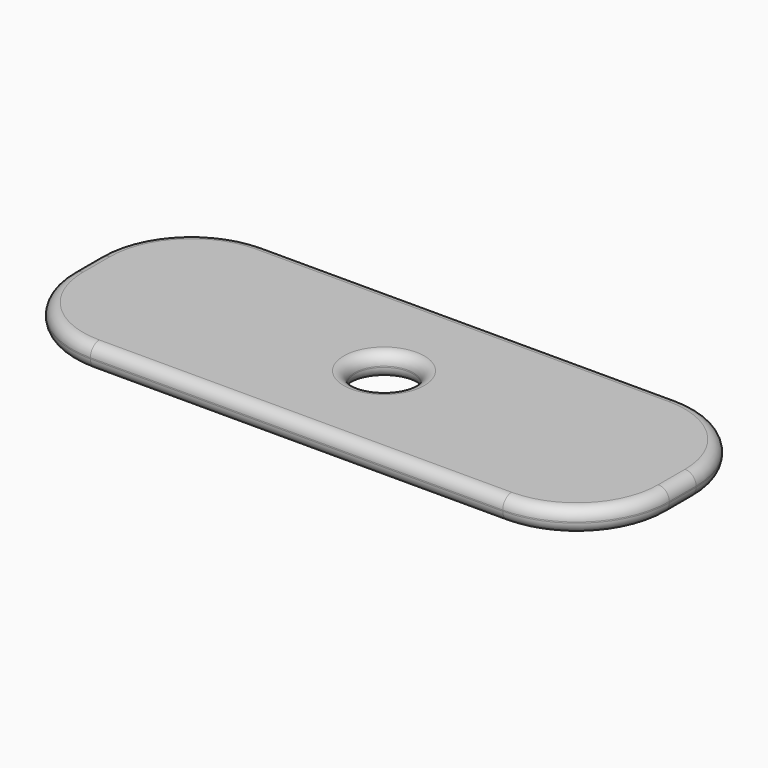
from build123d import *

# Parameters (mm, degrees)
F0_W     = 410
F0_H     = 150
F1_DEPTH = 16
F2_R     = 20
F3_DEPTH = 16.001
F4_R     = 63.5
F5_R     = 7.62


# Not quite as in the source:
# - a feature names something its author has since deleted; it is built from what else it names


with BuildPart() as f1:
    # F0 (on Top) → F1 (new body)
    with BuildSketch(Plane.XY):
        with Locations((-205, 75)):
            Rectangle(F0_W, F0_H)
    extrude(amount=F1_DEPTH)

    # F2 (on face) → F3 (cut, through all)
    with BuildSketch(Plane(origin=(0, 0, 0), x_dir=(1, 0, 0), z_dir=(0, 0, -1))):
        with Locations((-205, -75)):
            Circle(F2_R)
    extrude(amount=-F3_DEPTH, mode=Mode.SUBTRACT)

    # F4
    f4_edges = [f1.edges().sort_by_distance(p)[0] for p in [
        (-410, 150, 8),
        (-410, 0, 8),
        (0, 0, 8),
        (0, 150, 8),
    ]]
    fillet(f4_edges, radius=F4_R)

    # F5
    f5_edges = [f1.edges().sort_by_distance(p)[0] for p in [
        (-205, 0, 0),
        (-205, 0, 16),
        (-225, 75, 16),
        (-391.401281, 18.598719, 0),
        (-18.598719, 18.598719, 0),
        (-410, 75, 0),
        (0, 75, 0),
        (-391.401281, 131.401281, 0),
        (-18.598719, 131.401281, 0),
        (-205, 150, 0),
        (-225, 75, 0),
    ]]
    fillet(f5_edges, radius=F5_R)


solid = f1.part
